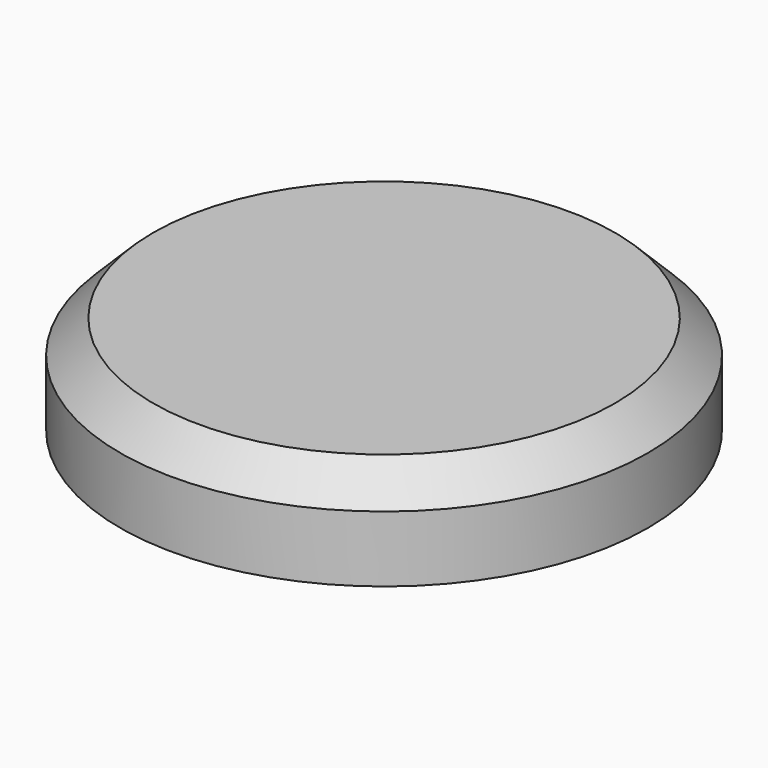
from build123d import *

# Parameters (mm, degrees)
F0_R     = 40
F1_DEPTH = 15
F2_SIZE  = 5
F3_R     = 25
F4_DEPTH = 10
F5_SIZE2 = 9.99999
F5_SIZE  = 24.99999


# Not quite as in the source:
# - a fillet or chamfer is up to 0.001 mm smaller than in the source, because OpenCascade refuses the exact size


with BuildPart() as f1:
    # F0 (on Top) → F1 (new body)
    with BuildSketch(Plane.XY):
        Circle(F0_R)
    extrude(amount=F1_DEPTH)

    # F2
    f2_edges = [f1.edges().sort_by_distance(p)[0] for p in [
        (-40, 0, 15),
    ]]
    chamfer(f2_edges, length=F2_SIZE)

    # F3 (on face) → F4 (cut)
    with BuildSketch(Plane(origin=(0, 0, 0), x_dir=(1, 0, 0), z_dir=(0, 0, -1))):
        Circle(F3_R)
    extrude(amount=-F4_DEPTH, mode=Mode.SUBTRACT)

    # F5 (size 25 and 10 in the source; OpenCascade refuses exactly that, so slightly less here)
    f5_edges = [f1.edges().sort_by_distance(p)[0] for p in [
        (-25, 0, 10),
    ]]
    f5_side = f1.faces().sort_by_distance((0, 0, 10))[0]
    chamfer(f5_edges, length=F5_SIZE, length2=F5_SIZE2, reference=f5_side)


solid = f1.part
